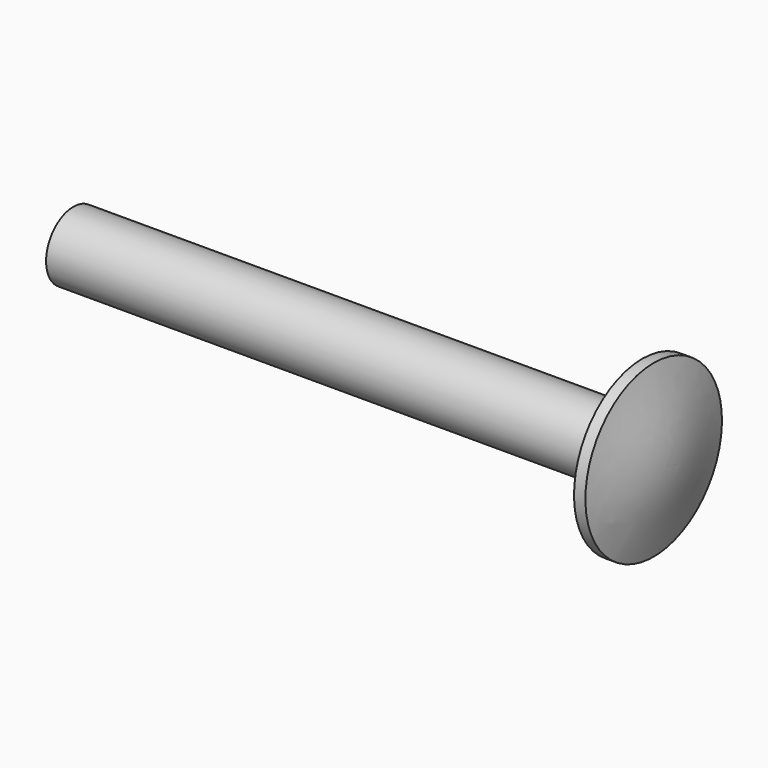
from build123d import *

# Parameters (mm, degrees)
F0_W = 100
F0_H = 6


# Not quite as in the source:
# - a feature of the source that left no trace in its solid (it failed there, or was rolled back) is left out


with BuildPart() as f1:
    # F0 (on Front) → F1 (revolve)
    with BuildSketch(Plane.XZ):
        with BuildLine():
            Line((88.4324429527, 10.4499064941), (88.4324429527, 1.4499064941))
            Line((88.4324429527, 1.4499064941), (88.4324429527, -4.5500935059))
            Line((88.4324429527, -4.5500935059), (93.4324429527, -4.5500935059))
            add(Edge.make_bspline(
                [(90.4324429527, 10.4499064941), (91.8025947904, 4.794743992), (93.5730556099, 0.3394810932), (93.4324429527, -4.5500935059)],
                knots=[0, 0, 0, 0, 15.2970585408, 15.2970585408, 15.2970585408, 15.2970585408], degree=3))
            Line((90.4324429527, 10.4499064941), (88.4324429527, 10.4499064941))
        make_face()
        with Locations((38.4324429527, -1.5500935059)):
            Rectangle(F0_W, F0_H)
    revolve(axis=Axis((38.4324429527, 0, -4.5500935059), (1, 0, 0)))


solid = f1.part
